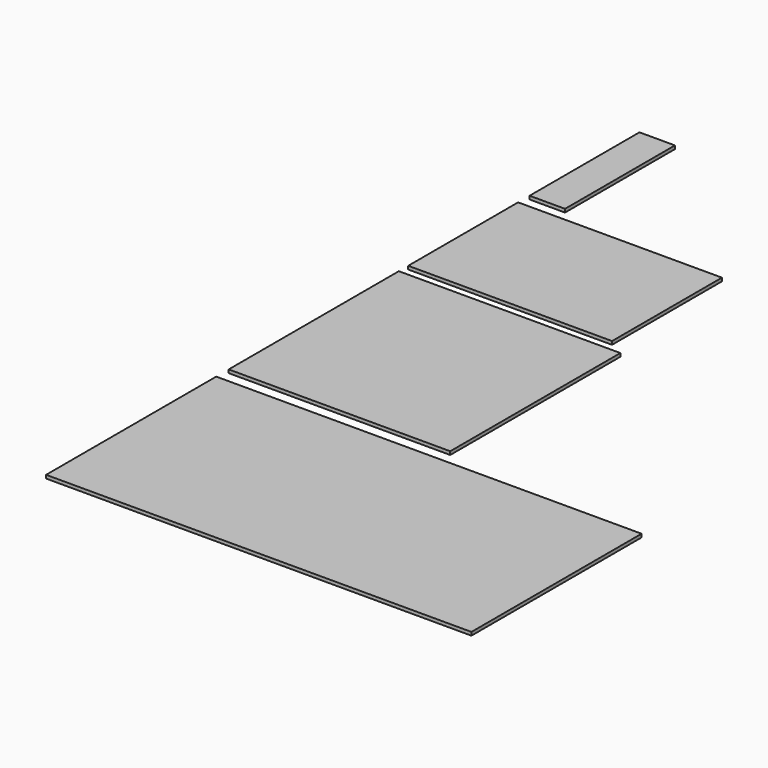
from build123d import *

# Parameters (mm, degrees)
F0_W     = 2438.4
F0_H     = 1219.2
F1_DEPTH = 19.05
F0_W_2   = 1270
F0_W_3   = 1168.4
F0_H_2   = 787.4
F0_W_4   = 203.2


# Not quite as in the source:
# - a length typed as a fraction of an inch, garbled in the dataset ("3 / 203.2 mm" for 3/8 in), is restored


with BuildPart() as f1:
    # F0 (on Top) → F1 (new body)
    with BuildSketch(Plane.XY):
        with Locations((1219.2, 609.6)):
            Rectangle(F0_W, F0_H)
    extrude(amount=F1_DEPTH)


with BuildPart() as f1b:
    # F0 (on Top) → F1, piece 2 (new body)
    with BuildSketch(Plane.XY):
        with Locations((635, 1918.174795723)):
            Rectangle(F0_W_2, F0_H)
    extrude(amount=F1_DEPTH)


with BuildPart() as f1c:
    # F0 (on Top) → F1, piece 3 (new body)
    with BuildSketch(Plane.XY):
        with Locations((584.2, 2988.8089931488)):
            Rectangle(F0_W_3, F0_H_2)
    extrude(amount=F1_DEPTH)


with BuildPart() as f1d:
    # F0 (on Top) → F1, piece 4 (new body)
    with BuildSketch(Plane.XY):
        with Locations((101.6, 3858.4023677826)):
            Rectangle(F0_W_4, F0_H_2)
    extrude(amount=F1_DEPTH)


solid = Compound([f1.part, f1b.part, f1c.part, f1d.part])
